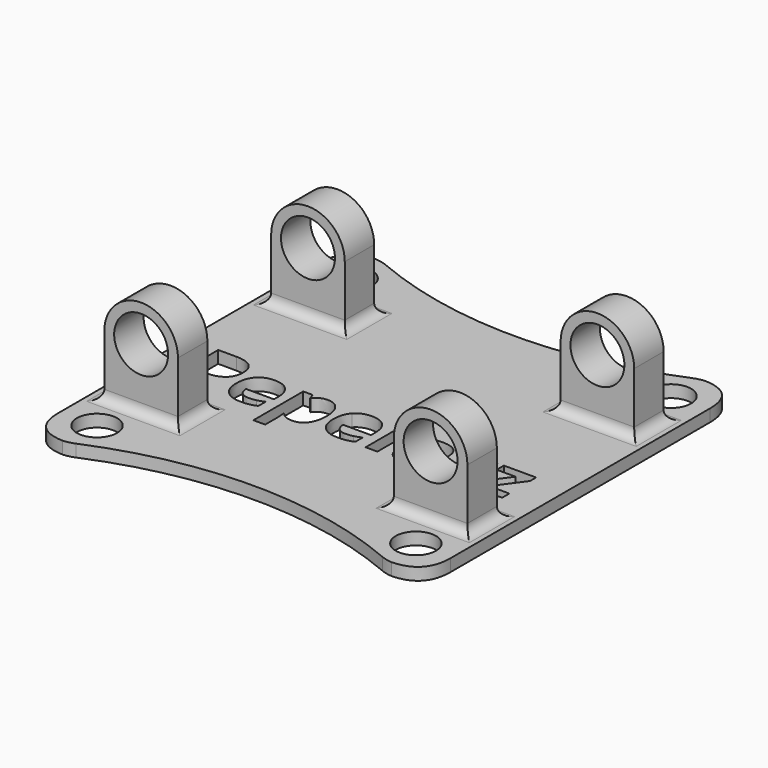
from build123d import *

# Parameters (mm, degrees)
F0_R        = 4.1
F0_W        = 2.4059684592
F0_H        = 12.2772556319
F1_DEPTH    = 2.5
F2_T1_DEPTH = 37.5
F2_T3_DEPTH = 9.7672372541
F3_R        = 5.5
F4_DEPTH    = 25
F5_DEPTH    = 17.5
F6_R        = 2


# Not quite as in the source:
# - a fillet or chamfer that OpenCascade refuses, or shapes differently, is made with other operations: its cross-section is extruded or revolved along the edge and cut away or added


with BuildPart() as f1:
    # F0 (on Top) → F1 (new body)
    with BuildSketch(Plane.XY):
        with BuildLine():
            Line((-32.5, 40), (-40, 40))
            Line((-40, 40), (-40, -40))
            Line((-40, -40), (-32.5, -40))
            ThreePointArc((-32.5, -40), (0, -33.1009575861), (32.5, -40))
            Line((32.5, -40), (40, -40))
            Line((40, -40), (40, 40))
            Line((40, 40), (32.5, 40))
            ThreePointArc((32.5, 40), (0, 33.1009575861), (-32.5, 40))
        make_face()
        with Locations((-32.5, -32.5)):
            Circle(F0_R, mode=Mode.SUBTRACT)
        with BuildLine():
            add(Edge.make_bspline(
                [(-26.8404028674, -1.0022764725), (-25.7485021763, -1.9060925359), (-25.7485021763, -3.6960522815)],
                knots=[0, 0, 0, 1, 1, 1], degree=2))
            add(Edge.make_bspline(
                [(-25.7485021763, -3.6960522815), (-25.7485021763, -5.5592261775), (-26.9123547048, -6.5450925819)],
                knots=[0, 0, 0, 1, 1, 1], degree=2))
            add(Edge.make_bspline(
                [(-26.9123547048, -6.5450925819), (-28.0762072334, -7.5309589862), (-30.2221392274, -7.5309589862)],
                knots=[0, 0, 0, 1, 1, 1], degree=2))
            Line((-30.2221392274, -7.5309589862), (-31.2698589657, -7.5309589862))
            Line((-31.2698589657, -7.5309589862), (-31.2698589657, -11.6334760337))
            Line((-31.2698589657, -11.6334760337), (-33.7162214389, -11.6334760337))
            Line((-33.7162214389, -11.6334760337), (-33.7162214389, -0.0984604091))
            Line((-33.7162214389, -0.0984604091), (-30.0327922868, -0.0984604091))
            add(Edge.make_bspline(
                [(-30.0327922868, -0.0984604091), (-27.9323035585, -0.0984604091), (-26.8404028674, -1.0022764725)],
                knots=[0, 0, 0, 1, 1, 1], degree=2))
        make_face(mode=Mode.SUBTRACT)
        with BuildLine():
            add(Edge.make_bspline(
                [(-18.01557312, -11.6385252854), (-18.7325668686, -11.7925274638), (-19.7676634775, -11.7925274638)],
                knots=[0, 0, 0, 1, 1, 1], degree=2))
            add(Edge.make_bspline(
                [(-19.7676634775, -11.7925274638), (-21.8959230905, -11.7925274638), (-23.0951203813, -10.6160518059)],
                knots=[0, 0, 0, 1, 1, 1], degree=2))
            add(Edge.make_bspline(
                [(-23.0951203813, -10.6160518059), (-24.2943176721, -9.439576148), (-24.2943176721, -7.2860702763)],
                knots=[0, 0, 0, 1, 1, 1], degree=2))
            add(Edge.make_bspline(
                [(-24.2943176721, -7.2860702763), (-24.2943176721, -5.0694487577), (-23.1860069128, -3.8588906505)],
                knots=[0, 0, 0, 1, 1, 1], degree=2))
            add(Edge.make_bspline(
                [(-23.1860069128, -3.8588906505), (-22.0776961535, -2.6483325433), (-20.1211111001, -2.6483325433)],
                knots=[0, 0, 0, 1, 1, 1], degree=2))
            add(Edge.make_bspline(
                [(-20.1211111001, -2.6483325433), (-18.2528879523, -2.6483325433), (-17.2114797787, -3.7124623497)],
                knots=[0, 0, 0, 1, 1, 1], degree=2))
            add(Edge.make_bspline(
                [(-17.2114797787, -3.7124623497), (-16.1700716052, -4.7765921562), (-16.1700716052, -6.6549138074)],
                knots=[0, 0, 0, 1, 1, 1], degree=2))
            Line((-16.1700716052, -6.6549138074), (-16.1700716052, -7.8238155877))
            Line((-16.1700716052, -7.8238155877), (-21.8580537023, -7.8238155877))
            add(Edge.make_bspline(
                [(-21.8580537023, -7.8238155877), (-21.8176596883, -8.8488136931), (-21.2496188664, -9.4244283927)],
                knots=[0, 0, 0, 1, 1, 1], degree=2))
            add(Edge.make_bspline(
                [(-21.2496188664, -9.4244283927), (-20.6815780444, -10.0000430923), (-19.656579939, -10.0000430923)],
                knots=[0, 0, 0, 1, 1, 1], degree=2))
            add(Edge.make_bspline(
                [(-19.656579939, -10.0000430923), (-18.8587981624, -10.0000430923), (-18.1493782914, -9.8346800975)],
                knots=[0, 0, 0, 1, 1, 1], degree=2))
            add(Edge.make_bspline(
                [(-18.1493782914, -9.8346800975), (-17.4399584205, -9.6693171026), (-16.6674229026, -9.3057709766)],
                knots=[0, 0, 0, 1, 1, 1], degree=2))
            Line((-16.6674229026, -9.3057709766), (-16.6674229026, -11.1689448726))
            add(Edge.make_bspline(
                [(-16.6674229026, -11.1689448726), (-17.2985793714, -11.484523107), (-18.01557312, -11.6385252854)],
                knots=[0, 0, 0, 1, 1, 1], degree=2))
        make_face(mode=Mode.SUBTRACT)
        with BuildLine():
            add(Edge.make_bspline(
                [(-7.5711958737, -11.2472082747), (-8.3361575139, -11.7925274638), (-9.3687294969, -11.7925274638)],
                knots=[0, 0, 0, 1, 1, 1], degree=2))
            add(Edge.make_bspline(
                [(-9.3687294969, -11.7925274638), (-10.9238990362, -11.7925274638), (-11.8075180925, -10.6640196975)],
                knots=[0, 0, 0, 1, 1, 1], degree=2))
            Line((-11.8075180925, -10.6640196975), (-11.9337493863, -10.6640196975))
            add(Edge.make_bspline(
                [(-11.9337493863, -10.6640196975), (-11.8075180925, -11.767281205), (-11.8075180925, -11.9414803904)],
                knots=[0, 0, 0, 1, 1, 1], degree=2))
            Line((-11.8075180925, -11.9414803904), (-11.8075180925, -15.51635063))
            Line((-11.8075180925, -15.51635063), (-14.2134865518, -15.51635063))
            Line((-14.2134865518, -15.51635063), (-14.2134865518, -2.8124332251))
            Line((-14.2134865518, -2.8124332251), (-12.2569014984, -2.8124332251))
            Line((-12.2569014984, -2.8124332251), (-11.9186016311, -3.9560887467))
            Line((-11.9186016311, -3.9560887467), (-11.8075180925, -3.9560887467))
            add(Edge.make_bspline(
                [(-11.8075180925, -3.9560887467), (-10.9617684243, -2.6483325433), (-9.3056138501, -2.6483325433)],
                knots=[0, 0, 0, 1, 1, 1], degree=2))
            add(Edge.make_bspline(
                [(-9.3056138501, -2.6483325433), (-7.7428704332, -2.6483325433), (-6.8592513768, -3.8551037117)],
                knots=[0, 0, 0, 1, 1, 1], degree=2))
            add(Edge.make_bspline(
                [(-6.8592513768, -3.8551037117), (-5.9756323205, -5.0618748801), (-5.9756323205, -7.2078068741)],
                knots=[0, 0, 0, 1, 1, 1], degree=2))
            add(Edge.make_bspline(
                [(-5.9756323205, -7.2078068741), (-5.9756323205, -8.6190727385), (-6.390933277, -9.6604809121)],
                knots=[0, 0, 0, 1, 1, 1], degree=2))
            add(Edge.make_bspline(
                [(-6.390933277, -9.6604809121), (-6.8062342335, -10.7018890856), (-7.5711958737, -11.2472082747)],
                knots=[0, 0, 0, 1, 1, 1], degree=2))
        make_face(mode=Mode.SUBTRACT)
        with BuildLine():
            add(Edge.make_bspline(
                [(1.7547721099, -11.6385252854), (1.0377783613, -11.7925274638), (0.0026817524, -11.7925274638)],
                knots=[0, 0, 0, 1, 1, 1], degree=2))
            add(Edge.make_bspline(
                [(0.0026817524, -11.7925274638), (-2.1255778605, -11.7925274638), (-3.3247751513, -10.6160518059)],
                knots=[0, 0, 0, 1, 1, 1], degree=2))
            add(Edge.make_bspline(
                [(-3.3247751513, -10.6160518059), (-4.5239724421, -9.439576148), (-4.5239724421, -7.2860702763)],
                knots=[0, 0, 0, 1, 1, 1], degree=2))
            add(Edge.make_bspline(
                [(-4.5239724421, -7.2860702763), (-4.5239724421, -5.0694487577), (-3.4156616828, -3.8588906505)],
                knots=[0, 0, 0, 1, 1, 1], degree=2))
            add(Edge.make_bspline(
                [(-3.4156616828, -3.8588906505), (-2.3073509236, -2.6483325433), (-0.3507658702, -2.6483325433)],
                knots=[0, 0, 0, 1, 1, 1], degree=2))
            add(Edge.make_bspline(
                [(-0.3507658702, -2.6483325433), (1.5174572776, -2.6483325433), (2.5588654512, -3.7124623497)],
                knots=[0, 0, 0, 1, 1, 1], degree=2))
            add(Edge.make_bspline(
                [(2.5588654512, -3.7124623497), (3.6002736248, -4.7765921562), (3.6002736248, -6.6549138074)],
                knots=[0, 0, 0, 1, 1, 1], degree=2))
            Line((3.6002736248, -6.6549138074), (3.6002736248, -7.8238155877))
            Line((3.6002736248, -7.8238155877), (-2.0877084724, -7.8238155877))
            add(Edge.make_bspline(
                [(-2.0877084724, -7.8238155877), (-2.0473144584, -8.8488136931), (-1.4792736364, -9.4244283927)],
                knots=[0, 0, 0, 1, 1, 1], degree=2))
            add(Edge.make_bspline(
                [(-1.4792736364, -9.4244283927), (-0.9112328145, -10.0000430923), (0.1137652909, -10.0000430923)],
                knots=[0, 0, 0, 1, 1, 1], degree=2))
            add(Edge.make_bspline(
                [(0.1137652909, -10.0000430923), (0.9115470675, -10.0000430923), (1.6209669385, -9.8346800975)],
                knots=[0, 0, 0, 1, 1, 1], degree=2))
            add(Edge.make_bspline(
                [(1.6209669385, -9.8346800975), (2.3303868095, -9.6693171026), (3.1029223273, -9.3057709766)],
                knots=[0, 0, 0, 1, 1, 1], degree=2))
            Line((3.1029223273, -9.3057709766), (3.1029223273, -11.1689448726))
            add(Edge.make_bspline(
                [(3.1029223273, -11.1689448726), (2.4717658585, -11.484523107), (1.7547721099, -11.6385252854)],
                knots=[0, 0, 0, 1, 1, 1], degree=2))
        make_face(mode=Mode.SUBTRACT)
        with Locations((32.5, -32.5)):
            Circle(F0_R, mode=Mode.SUBTRACT)
        with Locations((6.7598429078, -5.4948482177)):
            Rectangle(F0_W, F0_H, mode=Mode.SUBTRACT)
        with BuildLine():
            Line((17.7684740373, -11.6334760337), (16.0895978302, -11.6334760337))
            Line((16.0895978302, -11.6334760337), (15.6225420432, -10.4342787429))
            Line((15.6225420432, -10.4342787429), (15.5594263964, -10.4342787429))
            add(Edge.make_bspline(
                [(15.5594263964, -10.4342787429), (14.9535161863, -11.1992403831), (14.309736588, -11.4958839234)],
                knots=[0, 0, 0, 1, 1, 1], degree=2))
            add(Edge.make_bspline(
                [(14.309736588, -11.4958839234), (13.6659569898, -11.7925274638), (12.6333850068, -11.7925274638)],
                knots=[0, 0, 0, 1, 1, 1], degree=2))
            add(Edge.make_bspline(
                [(12.6333850068, -11.7925274638), (11.3634981915, -11.7925274638), (10.6338813135, -11.0654352117)],
                knots=[0, 0, 0, 1, 1, 1], degree=2))
            add(Edge.make_bspline(
                [(10.6338813135, -11.0654352117), (9.9042644355, -10.3383429596), (9.9042644355, -8.9977666198)],
                knots=[0, 0, 0, 1, 1, 1], degree=2))
            add(Edge.make_bspline(
                [(9.9042644355, -8.9977666198), (9.9042644355, -7.5940746331), (10.8863439011, -6.927573402)],
                knots=[0, 0, 0, 1, 1, 1], degree=2))
            add(Edge.make_bspline(
                [(10.8863439011, -6.927573402), (11.8684233666, -6.2610721709), (13.8477300529, -6.1903826464)],
                knots=[0, 0, 0, 1, 1, 1], degree=2))
            Line((13.8477300529, -6.1903826464), (15.3801779592, -6.1424147547))
            Line((15.3801779592, -6.1424147547), (15.3801779592, -5.7561469958))
            add(Edge.make_bspline(
                [(15.3801779592, -5.7561469958), (15.3801779592, -4.415570656), (14.006781483, -4.415570656)],
                knots=[0, 0, 0, 1, 1, 1], degree=2))
            add(Edge.make_bspline(
                [(14.006781483, -4.415570656), (12.9489632412, -4.415570656), (11.5200249958, -5.0543010025)],
                knots=[0, 0, 0, 1, 1, 1], degree=2))
            Line((11.5200249958, -5.0543010025), (10.724767845, -3.4284419387))
            add(Edge.make_bspline(
                [(10.724767845, -3.4284419387), (12.2471172479, -2.6306601621), (14.1001926404, -2.6306601621)],
                knots=[0, 0, 0, 1, 1, 1], degree=2))
            add(Edge.make_bspline(
                [(14.1001926404, -2.6306601621), (15.8750046308, -2.6306601621), (16.821739334, -3.4044579929)],
                knots=[0, 0, 0, 1, 1, 1], degree=2))
            add(Edge.make_bspline(
                [(16.821739334, -3.4044579929), (17.7684740373, -4.1782558237), (17.7684740373, -5.7561469958)],
                knots=[0, 0, 0, 1, 1, 1], degree=2))
            Line((17.7684740373, -5.7561469958), (17.7684740373, -11.6334760337))
        make_face(mode=Mode.SUBTRACT)
        with BuildLine():
            add(Edge.make_bspline(
                [(23.2014689211, -9.6289230886), (23.4892762709, -9.8738117985), (23.9639059354, -9.8738117985)],
                knots=[0, 0, 0, 1, 1, 1], degree=2))
            add(Edge.make_bspline(
                [(23.9639059354, -9.8738117985), (24.5950624043, -9.8738117985), (25.4786814606, -9.5986275781)],
                knots=[0, 0, 0, 1, 1, 1], degree=2))
            Line((25.4786814606, -9.5986275781), (25.4786814606, -11.3885873237))
            add(Edge.make_bspline(
                [(25.4786814606, -11.3885873237), (24.579914649, -11.7925274638), (23.2696338197, -11.7925274638)],
                knots=[0, 0, 0, 1, 1, 1], degree=2))
            add(Edge.make_bspline(
                [(23.2696338197, -11.7925274638), (21.825547819, -11.7925274638), (21.1666204655, -11.0616482729)],
                knots=[0, 0, 0, 1, 1, 1], degree=2))
            add(Edge.make_bspline(
                [(21.1666204655, -11.0616482729), (20.5076931121, -10.330769082), (20.5076931121, -8.871535326)],
                knots=[0, 0, 0, 1, 1, 1], degree=2))
            Line((20.5076931121, -8.871535326), (20.5076931121, -4.6200653519))
            Line((20.5076931121, -4.6200653519), (19.3564637129, -4.6200653519))
            Line((19.3564637129, -4.6200653519), (19.3564637129, -3.6026411241))
            Line((19.3564637129, -3.6026411241), (20.6818922975, -2.7972854699))
            Line((20.6818922975, -2.7972854699), (21.3761644132, -0.9341115739))
            Line((21.3761644132, -0.9341115739), (22.9136615713, -0.9341115739))
            Line((22.9136615713, -0.9341115739), (22.9136615713, -2.8124332251))
            Line((22.9136615713, -2.8124332251), (25.3827456774, -2.8124332251))
            Line((25.3827456774, -2.8124332251), (25.3827456774, -4.6200653519))
            Line((25.3827456774, -4.6200653519), (22.9136615713, -4.6200653519))
            Line((22.9136615713, -4.6200653519), (22.9136615713, -8.871535326))
            add(Edge.make_bspline(
                [(22.9136615713, -8.871535326), (22.9136615713, -9.3840343787), (23.2014689211, -9.6289230886)],
                knots=[0, 0, 0, 1, 1, 1], degree=2))
        make_face(mode=Mode.SUBTRACT)
        Polygon((33.3984328316, -9.7955483964), (33.3984328316, -11.6334760337), (26.4329900415, -11.6334760337), (26.4329900415, -10.2121116658), (30.5203593337, -4.6503608624), (26.6778787514, -4.6503608624), (26.6778787514, -2.8124332251), (33.2570537826, -2.8124332251), (33.2570537826, -4.375176642), (29.2807680289, -9.7955483964), align=None, mode=Mode.SUBTRACT)
        with Locations((-32.5, 32.5)):
            Circle(F0_R, mode=Mode.SUBTRACT)
        with Locations((32.5, 32.5)):
            Circle(F0_R, mode=Mode.SUBTRACT)
    extrude(amount=F1_DEPTH)

    # F2: fillet of radius 7 on 8 edges, made by hand

    # F2_s2 → F2_t1 (cut)
    with BuildSketch(Plane.XY.offset(-17.5)):
        with BuildLine():
            add(Edge.make_bspline(
                [(-40, -33), (-40, -40), (-33, -40)],
                knots=[0, 0, 0, 1, 1, 1], degree=2, weights=[1, 1, 1]))
            Line((-33, -40), (-40, -40))
            Line((-40, -40), (-40, -33))
        make_face()
        with BuildLine():
            add(Edge.make_bspline(
                [(33, -40), (40, -40), (40, -33)],
                knots=[0, 0, 0, 1, 1, 1], degree=2, weights=[1, 1, 1]))
            Line((40, -33), (40, -40))
            Line((40, -40), (33, -40))
        make_face()
        with BuildLine():
            add(Edge.make_bspline(
                [(-33, 40), (-40, 40), (-40, 33)],
                knots=[0, 0, 0, 1, 1, 1], degree=2, weights=[1, 1, 1]))
            Line((-40, 33), (-40, 40))
            Line((-40, 40), (-33, 40))
        make_face()
        with BuildLine():
            add(Edge.make_bspline(
                [(40, 33), (40, 40), (33, 40)],
                knots=[0, 0, 0, 1, 1, 1], degree=2, weights=[1, 1, 1]))
            Line((33, 40), (40, 40))
            Line((40, 40), (40, 33))
        make_face()
    extrude(amount=F2_T1_DEPTH, mode=Mode.SUBTRACT)

    # F2_s4 → F2_t3 (cut)
    with BuildSketch(Plane.XY.offset(-3.633618627)):
        with BuildLine():
            add(Edge.make_bspline(
                [(-33.9534474508, -40), (-32.5311089102, -40), (-31.2215608743, -39.4449046334)],
                knots=[0, 0, 0, 1, 1, 1], degree=2, weights=[1, 1, 1]))
            ThreePointArc((-31.2215608743, -39.4449046334), (-31.8619893099, -39.7196681642), (-32.5, -40))
            Line((-32.5, -40), (-33.9534474508, -40))
        make_face()
        with BuildLine():
            add(Edge.make_bspline(
                [(31.2215608743, -39.4449046334), (32.5311089102, -40), (33.9534474508, -40)],
                knots=[0, 0, 0, 1, 1, 1], degree=2, weights=[1, 1, 1]))
            Line((33.9534474508, -40), (32.5, -40))
            ThreePointArc((32.5, -40), (31.8619893099, -39.7196681642), (31.2215608743, -39.4449046334))
        make_face()
        with BuildLine():
            add(Edge.make_bspline(
                [(31.2215608743, 39.4449046334), (32.5311089102, 40), (33.9534474508, 40)],
                knots=[0, 0, 0, 1, 1, 1], degree=2, weights=[1, 1, 1]))
            Line((33.9534474508, 40), (32.5, 40))
            ThreePointArc((32.5, 40), (31.8619893099, 39.7196681642), (31.2215608743, 39.4449046334))
        make_face()
        with BuildLine():
            add(Edge.make_bspline(
                [(-31.2215608743, 39.4449046334), (-32.5311089102, 40), (-33.9534474508, 40)],
                knots=[0, 0, 0, 1, 1, 1], degree=2, weights=[1, 1, 1]))
            Line((-33.9534474508, 40), (-32.5, 40))
            ThreePointArc((-32.5, 40), (-31.8619893099, 39.7196681642), (-31.2215608743, 39.4449046334))
        make_face()
    extrude(amount=F2_T3_DEPTH, mode=Mode.SUBTRACT)

    # F3 (on Front) → F4 (join, symmetric)
    with BuildSketch(Plane.XZ):
        with BuildLine():
            ThreePointArc((-37, 15), (-29.5, 7.5), (-22, 15))
            ThreePointArc((-22, 15), (-29.5, 22.5), (-37, 15))
        make_face()
        with Locations((-29.5, 15)):
            Circle(F3_R, mode=Mode.SUBTRACT)
        with BuildLine():
            Line((-22, 2.5), (-22, 15))
            ThreePointArc((-22, 15), (-29.5, 7.5), (-37, 15))
            Line((-37, 15), (-37, 2.5))
            Line((-37, 2.5), (-22, 2.5))
        make_face()
        with BuildLine():
            ThreePointArc((22, 15), (29.5, 7.5), (37, 15))
            ThreePointArc((37, 15), (29.5, 22.5), (22, 15))
        make_face()
        with Locations((29.5, 15)):
            Circle(F3_R, mode=Mode.SUBTRACT)
        with BuildLine():
            Line((37, 2.5), (37, 15))
            ThreePointArc((37, 15), (29.5, 7.5), (22, 15))
            Line((22, 15), (22, 2.5))
            Line((22, 2.5), (37, 2.5))
        make_face()
    extrude(amount=F4_DEPTH, both=True)

    # F3 (on Front) → F5 (cut, symmetric)
    with BuildSketch(Plane.XZ):
        with BuildLine():
            ThreePointArc((-37, 15), (-29.5, 7.5), (-22, 15))
            ThreePointArc((-22, 15), (-29.5, 22.5), (-37, 15))
        make_face()
        with Locations((-29.5, 15)):
            Circle(F3_R, mode=Mode.SUBTRACT)
        with BuildLine():
            Line((-22, 2.5), (-22, 15))
            ThreePointArc((-22, 15), (-29.5, 7.5), (-37, 15))
            Line((-37, 15), (-37, 2.5))
            Line((-37, 2.5), (-22, 2.5))
        make_face()
        with BuildLine():
            ThreePointArc((22, 15), (29.5, 7.5), (37, 15))
            ThreePointArc((37, 15), (29.5, 22.5), (22, 15))
        make_face()
        with Locations((29.5, 15)):
            Circle(F3_R, mode=Mode.SUBTRACT)
        with BuildLine():
            Line((37, 2.5), (37, 15))
            ThreePointArc((37, 15), (29.5, 7.5), (22, 15))
            Line((22, 15), (22, 2.5))
            Line((22, 2.5), (37, 2.5))
        make_face()
    extrude(amount=F5_DEPTH, both=True, mode=Mode.SUBTRACT)

    # F6
    f6_edges = [f1.edges().sort_by_distance(p)[0] for p in [
        (-37, -21.25, 2.5),
        (-22, -21.25, 2.5),
        (22, -21.25, 2.5),
        (37, -21.25, 2.5),
        (37, 21.25, 2.5),
        (22, 21.25, 2.5),
        (-22, 21.25, 2.5),
        (-37, 21.25, 2.5),
        (-29.5, 17.5, 2.5),
        (-29.5, -25, 2.5),
        (-29.5, -17.5, 2.5),
        (-29.5, 25, 2.5),
        (29.5, 25, 2.5),
        (29.5, 17.5, 2.5),
        (29.5, -25, 2.5),
        (29.5, -17.5, 2.5),
    ]]
    fillet(f6_edges, radius=F6_R)


solid = f1.part
